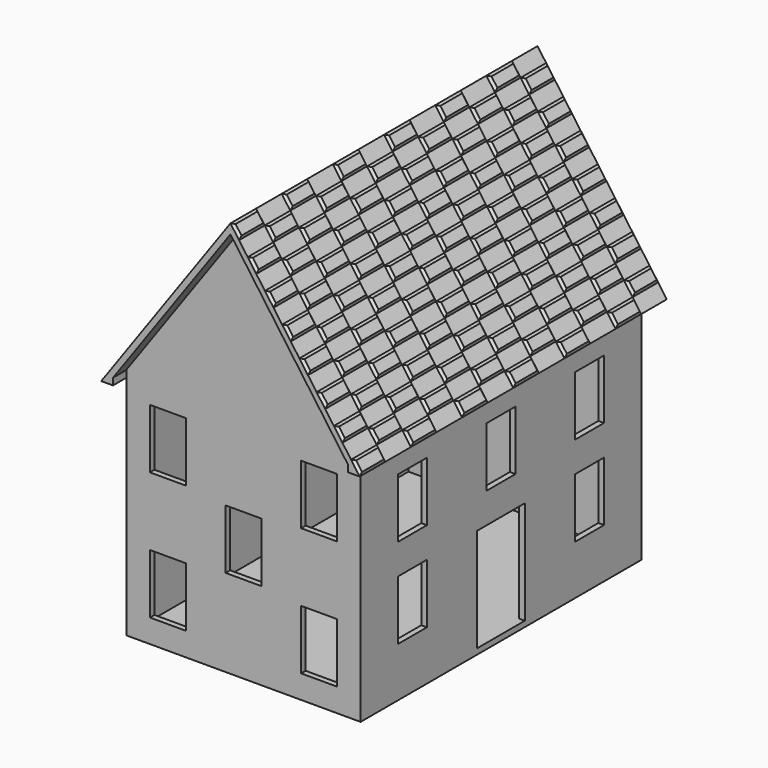
from build123d import *

# Parameters (mm, degrees)
F1_W      = 100
F1_H      = 150
F2_DEPTH  = 100
F3_T      = -2.4
F5_DEPTH  = 2.4
F7_DEPTH  = 2.4
F8_W      = 15.4
F8_H      = 25.4
F9_DEPTH  = 2.4
F10_W     = 15.4
F10_H     = 25.4
F10_W_2   = 25.4
F10_H_2   = 44.2
F11_DEPTH = 2.4
F15_DEPTH = 164
F16_W     = 13.66666672
F16_H     = 6.330327
F17_DEPTH = 1
F17_TAPER = 45
F16_W_2   = 13.6666666
F16_H_2   = 6.333333
F18_DEPTH = 1
F18_TAPER = 45


# Not quite as in the source:
# - ends of sketch curves that miss each other by under 0.0002 mm in the source are joined


with BuildPart() as f2:
    # F1 (on Top) → F2 (new body)
    with BuildSketch(Plane.XY):
        Rectangle(F1_W, F1_H)
    extrude(amount=F2_DEPTH)

    # F3
    f3_openings = [f2.faces().sort_by_distance(p)[0] for p in [
        (0, 0, 100),
    ]]
    offset(amount=F3_T, openings=f3_openings)

    # F4 (on face) → F5 (join)
    with BuildSketch(Plane.XZ.offset(75)):
        Polygon((0, 170), (-50, 100), (50, 100), align=None)
    extrude(amount=-F5_DEPTH)

    # F6 (on face) → F7 (join)
    with BuildSketch(Plane(origin=(0, 75, 0), x_dir=(-1, 0, 0), z_dir=(0, 1, 0))):
        Polygon((-50, 100), (50, 100), (0, 170), align=None)
    extrude(amount=-F7_DEPTH)

    # F8 (on face) → F9 (cut, through all)
    with BuildSketch(Plane.XZ.offset(75)):
        with Locations((-32.3, 77.3)):
            Rectangle(F8_W, F8_H)
        with Locations((32.3, 77.3)):
            Rectangle(F8_W, F8_H)
        with Locations((0, 50)):
            Rectangle(F8_W, F8_H)
        with Locations((32.3, 22.7)):
            Rectangle(F8_W, F8_H)
        with Locations((-32.3, 22.7)):
            Rectangle(F8_W, F8_H)
    extrude(amount=-F9_DEPTH, mode=Mode.SUBTRACT)

    # F10 (on face) → F11 (cut, through all)
    with BuildSketch(Plane.YZ.offset(50)):
        with Locations((-47.3, 72.3)):
            Rectangle(F10_W, F10_H)
        with Locations((47.3, 72.3)):
            Rectangle(F10_W, F10_H)
        with Locations((-47.3, 33.9)):
            Rectangle(F10_W, F10_H)
        with Locations((47.3, 33.9)):
            Rectangle(F10_W, F10_H)
        with Locations((0, 72.3)):
            Rectangle(F10_W, F10_H)
        with Locations((0, 24.5)):
            Rectangle(F10_W_2, F10_H_2)
    extrude(amount=-F11_DEPTH, mode=Mode.SUBTRACT)


with BuildPart() as f15:
    # F14 (on offset) → F15 (new body)
    with BuildSketch(Plane.XZ.offset(82)):
        Polygon((0, 174.1291161282), (-55.2176284033, 96.8244363635), (-50.2, 96.8244363635), (-50.2, 99.72), (-50, 100), (0, 170), (50, 100), (50.2, 99.72), (50.2, 96.8244363635), (55.2176284033, 96.8244363635), align=None)
    extrude(amount=-F15_DEPTH)

    # F16 (on face) → F17 (join)
    with BuildSketch(Plane(origin=(82.3583657363, 0, 58.8274040974), x_dir=(0, 1, 0), z_dir=(0.8137334712, 0, 0.5812381937))):
        Polygon((-68.3333334, 97.3693571051), (-68.3333334, 91.0400501051), (-68.3333334, 91.0390301051), (-54.66666668, 91.0390301051), (-54.66666668, 91.0400501051), (-54.66666668, 97.3693571051), align=None)
        Polygon((-68.3333334, 84.7053571051), (-68.3333334, 78.3763901051), (-68.3333334, 78.3750301051), (-54.66666668, 78.3750301051), (-54.66666668, 78.3763901051), (-54.66666668, 84.7053571051), align=None)
        Polygon((-68.3333334, 72.0413571051), (-68.3333334, 65.7127301051), (-68.3333334, 65.7110301051), (-54.66666668, 65.7110301051), (-54.66666668, 65.7127301051), (-54.66666668, 72.0413571051), align=None)
        Polygon((-68.3333334, 59.3773571051), (-68.3333334, 53.0490701051), (-68.3333334, 53.0470301051), (-54.66666668, 53.0470301051), (-54.66666668, 53.0490701051), (-54.66666668, 59.3773571051), align=None)
        with Locations((-34.16666704, 132.1961936051)):
            Rectangle(F16_W, F16_H)
        Polygon((-41.0000004, 122.6973571051), (-41.0000004, 116.3673701051), (-41.00000008, 116.3670301051), (-27.33333368, 116.3670301051), (-27.33333336, 116.3673701051), (-27.33333368, 122.6973571051), align=None)
        Polygon((-41.0000004, 110.0333571051), (-41.0000004, 103.7037101051), (-41.00000008, 103.7030301051), (-27.33333368, 103.7030301051), (-27.33333336, 103.7037101051), (-27.33333368, 110.0333571051), align=None)
        Polygon((-41.0000004, 97.3693571051), (-41.0000004, 91.0400501051), (-41.00000008, 91.0390301051), (-27.33333368, 91.0390301051), (-27.33333336, 91.0400501051), (-27.33333368, 97.3693571051), align=None)
        Polygon((-41.0000004, 84.7053571051), (-41.0000004, 78.3763901051), (-41.00000008, 78.3750301051), (-27.33333368, 78.3750301051), (-27.33333336, 78.3763901051), (-27.33333368, 84.7053571051), align=None)
        Polygon((-41.0000004, 72.0413571051), (-41.0000004, 65.7127301051), (-41.00000008, 65.7110301051), (-27.33333368, 65.7110301051), (-27.33333336, 65.7127301051), (-27.33333368, 72.0413571051), align=None)
        Polygon((-41.0000004, 59.3773571051), (-41.0000004, 53.0490701051), (-41.00000008, 53.0470301051), (-27.33333368, 53.0470301051), (-27.33333336, 53.0490701051), (-27.33333368, 59.3773571051), align=None)
        with Locations((-6.83333404, 132.1961936051)):
            Rectangle(F16_W, F16_H)
        Polygon((-13.6666674, 122.6973571051), (-13.6666674, 116.3673701051), (-13.66666676, 116.3670301051), (-6.8e-07, 116.3670301051), (-4e-08, 116.3673701051), (-6.8e-07, 122.6973571051), align=None)
        Polygon((-13.6666674, 110.0333571051), (-13.6666674, 103.7037101051), (-13.66666676, 103.7030301051), (-6.8e-07, 103.7030301051), (-4e-08, 103.7037101051), (-6.8e-07, 110.0333571051), align=None)
        Polygon((-13.6666674, 97.3693571051), (-13.6666674, 91.0400501051), (-13.66666676, 91.0390301051), (-6.8e-07, 91.0390301051), (-4e-08, 91.0400501051), (-6.8e-07, 97.3693571051), align=None)
        Polygon((-13.6666674, 84.7053571051), (-13.6666674, 78.3763901051), (-13.66666676, 78.3750301051), (-6.8e-07, 78.3750301051), (-4e-08, 78.3763901051), (-6.8e-07, 84.7053571051), align=None)
        Polygon((-13.6666674, 72.0413571051), (-13.6666674, 65.7127301051), (-13.66666676, 65.7110301051), (-6.8e-07, 65.7110301051), (-4e-08, 65.7127301051), (-6.8e-07, 72.0413571051), align=None)
        Polygon((-13.6666674, 59.3773571051), (-13.6666674, 53.0490701051), (-13.66666676, 53.0470301051), (-6.8e-07, 53.0470301051), (-4e-08, 53.0490701051), (-6.8e-07, 59.3773571051), align=None)
        with Locations((20.49999896, 132.1961936051)):
            Rectangle(F16_W, F16_H)
        Polygon((13.6666656, 122.6973571051), (13.6666656, 116.3673701051), (13.66666656, 116.3670301051), (27.33333232, 116.3670301051), (27.33333328, 116.3673701051), (27.33333232, 122.6973571051), align=None)
        Polygon((13.6666656, 110.0333571051), (13.6666656, 103.7037101051), (13.66666656, 103.7030301051), (27.33333232, 103.7030301051), (27.33333328, 103.7037101051), (27.33333232, 110.0333571051), align=None)
        Polygon((13.6666656, 97.3693571051), (13.6666656, 91.0400501051), (13.66666656, 91.0390301051), (27.33333232, 91.0390301051), (27.33333328, 91.0400501051), (27.33333232, 97.3693571051), align=None)
        Polygon((13.6666656, 84.7053571051), (13.6666656, 78.3763901051), (13.66666656, 78.3750301051), (27.33333232, 78.3750301051), (27.33333328, 78.3763901051), (27.33333232, 84.7053571051), align=None)
        Polygon((13.6666656, 72.0413571051), (13.6666656, 65.7127301051), (13.66666656, 65.7110301051), (27.33333232, 65.7110301051), (27.33333328, 65.7127301051), (27.33333232, 72.0413571051), align=None)
        Polygon((27.33333328, 53.0470301051), (27.33333328, 53.0490701051), (27.33333232, 59.3773571051), (13.6666656, 59.3773571051), (13.6666656, 53.0490701051), (13.66666656, 53.0470301051), align=None)
        with Locations((47.83333196, 132.1961936051)):
            Rectangle(F16_W, F16_H)
        Polygon((54.6666666, 116.3670301051), (54.6666666, 116.3673701051), (54.66666532, 122.6973571051), (40.9999986, 122.6973571051), (40.9999986, 116.3673701051), (40.99999988, 116.3670301051), align=None)
        Polygon((54.6666666, 103.7030301051), (54.6666666, 103.7037101051), (54.66666532, 110.0333571051), (40.9999986, 110.0333571051), (40.9999986, 103.7037101051), (40.99999988, 103.7030301051), align=None)
        Polygon((54.6666666, 91.0390301051), (54.6666666, 91.0400501051), (54.66666532, 97.3693571051), (40.9999986, 97.3693571051), (40.9999986, 91.0400501051), (40.99999988, 91.0390301051), align=None)
        Polygon((54.6666666, 78.3750301051), (54.6666666, 78.3763901051), (54.66666532, 84.7053571051), (40.9999986, 84.7053571051), (40.9999986, 78.3763901051), (40.99999988, 78.3750301051), align=None)
        Polygon((54.6666666, 65.7110301051), (54.6666666, 65.7127301051), (54.66666532, 72.0413571051), (40.9999986, 72.0413571051), (40.9999986, 65.7127301051), (40.99999988, 65.7110301051), align=None)
        Polygon((54.6666666, 53.0470301051), (54.6666666, 53.0490701051), (54.66666532, 59.3773571051), (40.9999986, 59.3773571051), (40.9999986, 53.0490701051), (40.99999988, 53.0470301051), align=None)
        with Locations((-61.50000004, 132.1961936051)):
            Rectangle(F16_W, F16_H)
        Polygon((-68.3333334, 110.0333571051), (-68.3333334, 103.7037101051), (-68.3333334, 103.7030301051), (-54.66666668, 103.7030301051), (-54.66666668, 103.7037101051), (-54.66666668, 110.0333571051), align=None)
        Polygon((-68.3333334, 122.6973571051), (-68.3333334, 116.3673701051), (-68.3333334, 116.3670301051), (-54.66666668, 116.3670301051), (-54.66666668, 116.3673701051), (-54.66666668, 122.6973571051), align=None)
        Polygon((68.3333316, 53.0470301051), (81.99999832, 53.0470301051), (81.99999832, 59.3773571051), (68.3333316, 59.3773571051), (68.3333316, 53.0490701051), align=None)
        Polygon((68.3333316, 65.7110301051), (81.99999832, 65.7110301051), (81.99999832, 72.0413571051), (68.3333316, 72.0413571051), (68.3333316, 65.7127301051), align=None)
        Polygon((81.99999832, 78.3750301051), (81.99999832, 84.7053571051), (68.3333316, 84.7053571051), (68.3333316, 78.3763901051), (68.3333332, 78.3750301051), align=None)
        Polygon((81.99999832, 91.0390301051), (81.99999832, 97.3693571051), (68.3333316, 97.3693571051), (68.3333316, 91.0400501051), (68.3333332, 91.0390301051), align=None)
        Polygon((81.99999832, 103.7030301051), (81.99999832, 110.0333571051), (68.3333316, 110.0333571051), (68.3333316, 103.7037101051), (68.3333332, 103.7030301051), align=None)
        Polygon((81.99999832, 116.3670301051), (81.99999832, 122.6973571051), (68.3333316, 122.6973571051), (68.3333316, 116.3673701051), (68.3333332, 116.3670301051), align=None)
        with Locations((75.16666496, 132.1961936051)):
            Rectangle(F16_W, F16_H)
    extrude(amount=F17_DEPTH, taper=F17_TAPER)

    # F16 (on face) → F18 (join)
    with BuildSketch(Plane(origin=(82.3583657363, 0, 58.8274040974), x_dir=(0, 1, 0), z_dir=(0.8137334712, 0, 0.5812381937))):
        with Locations((-75.1666667, 138.5280236051)):
            Rectangle(F16_W_2, F16_H_2)
        with Locations((-75.1666667, 125.8643636051)):
            Rectangle(F16_W_2, F16_H_2)
        Polygon((-68.3333334, 116.3673701051), (-82, 116.3673701051), (-82, 110.0340371051), (-68.3333334, 110.0340371051), (-68.3333334, 116.3670301051), align=None)
        Polygon((-68.3333334, 103.7037101051), (-82, 103.7037101051), (-82, 97.3703771051), (-68.3333334, 97.3703771051), (-68.3333334, 103.7030301051), align=None)
        Polygon((-68.3333334, 91.0400501051), (-82, 91.0400501051), (-82, 84.7067171051), (-68.3333334, 84.7067171051), (-68.3333334, 91.0390301051), align=None)
        Polygon((-68.3333334, 78.3763901051), (-82, 78.3763901051), (-82, 72.0430571051), (-68.3333334, 72.0430571051), (-68.3333334, 78.3750301051), align=None)
        Polygon((-68.3333334, 65.7127301051), (-82, 65.7127301051), (-82, 59.3793971051), (-68.3333334, 59.3793971051), (-68.3333334, 65.7110301051), align=None)
        Polygon((-68.3333334, 53.0490701051), (-82, 53.0490701051), (-82, 46.7157371051), (-68.3333334, 46.7157371051), (-68.3333334, 53.0470301051), align=None)
        with Locations((-47.83333338, 138.5280236051)):
            Rectangle(F16_W_2, F16_H_2)
        with Locations((-47.83333338, 125.8643636051)):
            Rectangle(F16_W_2, F16_H_2)
        with Locations((-20.50000006, 125.8643636051)):
            Rectangle(F16_W_2, F16_H_2)
        with Locations((-20.50000006, 138.5280236051)):
            Rectangle(F16_W_2, F16_H_2)
        with Locations((6.83333326, 138.5280236051)):
            Rectangle(F16_W_2, F16_H_2)
        with Locations((6.83333326, 125.8643636051)):
            Rectangle(F16_W_2, F16_H_2)
        with Locations((34.16666658, 138.5280236051)):
            Rectangle(F16_W_2, F16_H_2)
        with Locations((34.16666658, 125.8643636051)):
            Rectangle(F16_W_2, F16_H_2)
        with Locations((61.4999999, 138.5280236051)):
            Rectangle(F16_W_2, F16_H_2)
        with Locations((61.4999999, 125.8643636051)):
            Rectangle(F16_W_2, F16_H_2)
        Polygon((-54.66666668, 116.3673701051), (-54.66666668, 116.3670301051), (-54.66666668, 110.0340371051), (-41.00000008, 110.0340371051), (-41.00000008, 116.3670301051), (-41.00000008, 116.3673701051), align=None)
        Polygon((-27.33333336, 116.3673701051), (-27.33333336, 116.3670301051), (-27.33333336, 110.0340371051), (-13.66666676, 110.0340371051), (-13.66666676, 116.3670301051), (-13.66666676, 116.3673701051), align=None)
        Polygon((-4e-08, 116.3673701051), (-4e-08, 116.3670301051), (-4e-08, 110.0340371051), (13.66666656, 110.0340371051), (13.66666656, 116.3670301051), (13.66666656, 116.3673701051), align=None)
        Polygon((27.33333328, 116.3673701051), (27.33333328, 116.3670301051), (27.33333328, 110.0340371051), (40.99999988, 110.0340371051), (40.99999988, 116.3670301051), (40.99999988, 116.3673701051), align=None)
        Polygon((68.3333332, 116.3670301051), (68.3333332, 116.3673701051), (54.6666666, 116.3673701051), (54.6666666, 116.3670301051), (54.6666666, 110.0340371051), (68.3333332, 110.0340371051), align=None)
        Polygon((68.3333332, 103.7030301051), (68.3333332, 103.7037101051), (54.6666666, 103.7037101051), (54.6666666, 103.7030301051), (54.6666666, 97.3703771051), (68.3333332, 97.3703771051), align=None)
        Polygon((27.33333328, 103.7037101051), (27.33333328, 103.7030301051), (27.33333328, 97.3703771051), (40.99999988, 97.3703771051), (40.99999988, 103.7030301051), (40.99999988, 103.7037101051), align=None)
        Polygon((-4e-08, 103.7037101051), (-4e-08, 103.7030301051), (-4e-08, 97.3703771051), (13.66666656, 97.3703771051), (13.66666656, 103.7030301051), (13.66666656, 103.7037101051), align=None)
        Polygon((-27.33333336, 103.7037101051), (-27.33333336, 103.7030301051), (-27.33333336, 97.3703771051), (-13.66666676, 97.3703771051), (-13.66666676, 103.7030301051), (-13.66666676, 103.7037101051), align=None)
        Polygon((-54.66666668, 103.7037101051), (-54.66666668, 103.7030301051), (-54.66666668, 97.3703771051), (-41.00000008, 97.3703771051), (-41.00000008, 103.7030301051), (-41.00000008, 103.7037101051), align=None)
        Polygon((-54.66666668, 91.0400501051), (-54.66666668, 91.0390301051), (-54.66666668, 84.7067171051), (-41.00000008, 84.7067171051), (-41.00000008, 91.0390301051), (-41.00000008, 91.0400501051), align=None)
        Polygon((-27.33333336, 91.0400501051), (-27.33333336, 91.0390301051), (-27.33333336, 84.7067171051), (-13.66666676, 84.7067171051), (-13.66666676, 91.0390301051), (-13.66666676, 91.0400501051), align=None)
        Polygon((-4e-08, 91.0400501051), (-4e-08, 91.0390301051), (-4e-08, 84.7067171051), (13.66666656, 84.7067171051), (13.66666656, 91.0390301051), (13.66666656, 91.0400501051), align=None)
        Polygon((27.33333328, 91.0400501051), (27.33333328, 91.0390301051), (27.33333328, 84.7067171051), (40.99999988, 84.7067171051), (40.99999988, 91.0390301051), (40.99999988, 91.0400501051), align=None)
        Polygon((68.3333332, 91.0390301051), (68.3333332, 91.0400501051), (54.6666666, 91.0400501051), (54.6666666, 91.0390301051), (54.6666666, 84.7067171051), (68.3333332, 84.7067171051), align=None)
        Polygon((-54.66666668, 78.3763901051), (-54.66666668, 78.3750301051), (-54.66666668, 72.0430571051), (-41.00000008, 72.0430571051), (-41.00000008, 78.3750301051), (-41.00000008, 78.3763901051), align=None)
        Polygon((-27.33333336, 78.3763901051), (-27.33333336, 78.3750301051), (-27.33333336, 72.0430571051), (-13.66666676, 72.0430571051), (-13.66666676, 78.3750301051), (-13.66666676, 78.3763901051), align=None)
        Polygon((-4e-08, 78.3763901051), (-4e-08, 78.3750301051), (-4e-08, 72.0430571051), (13.66666656, 72.0430571051), (13.66666656, 78.3750301051), (13.66666656, 78.3763901051), align=None)
        Polygon((27.33333328, 78.3763901051), (27.33333328, 78.3750301051), (27.33333328, 72.0430571051), (40.99999988, 72.0430571051), (40.99999988, 78.3750301051), (40.99999988, 78.3763901051), align=None)
        Polygon((68.3333332, 78.3750301051), (68.3333332, 78.3763901051), (54.6666666, 78.3763901051), (54.6666666, 78.3750301051), (54.6666666, 72.0430571051), (68.3333332, 72.0430571051), align=None)
        Polygon((-54.66666668, 65.7127301051), (-54.66666668, 65.7110301051), (-54.66666668, 59.3793971051), (-41.00000008, 59.3793971051), (-41.00000008, 65.7110301051), (-41.00000008, 65.7127301051), align=None)
        Polygon((-27.33333336, 65.7127301051), (-27.33333336, 65.7110301051), (-27.33333336, 59.3793971051), (-13.66666676, 59.3793971051), (-13.66666676, 65.7110301051), (-13.66666676, 65.7127301051), align=None)
        Polygon((-4e-08, 65.7127301051), (-4e-08, 65.7110301051), (-4e-08, 59.3793971051), (13.66666656, 59.3793971051), (13.66666656, 65.7110301051), (13.66666656, 65.7127301051), align=None)
        Polygon((40.99999988, 59.3793971051), (40.99999988, 65.7110301051), (40.99999988, 65.7127301051), (27.33333328, 65.7127301051), (27.33333328, 65.7110301051), (27.33333328, 59.3793971051), align=None)
        Polygon((68.3333332, 59.3793971051), (68.3333332, 65.7110301051), (68.3333332, 65.7127301051), (54.6666666, 65.7127301051), (54.6666666, 65.7110301051), (54.6666666, 59.3793971051), align=None)
        Polygon((68.3333332, 46.7157371051), (68.3333332, 53.0470301051), (68.3333332, 53.0490701051), (54.6666666, 53.0490701051), (54.6666666, 53.0470301051), (54.6666666, 46.7157371051), align=None)
        Polygon((40.99999988, 46.7157371051), (40.99999988, 53.0470301051), (40.99999988, 53.0490701051), (27.33333328, 53.0490701051), (27.33333328, 53.0470301051), (27.33333328, 46.7157371051), align=None)
        Polygon((-4e-08, 53.0490701051), (-4e-08, 53.0470301051), (-4e-08, 46.7157371051), (13.66666656, 46.7157371051), (13.66666656, 53.0470301051), (13.66666656, 53.0490701051), align=None)
        Polygon((-27.33333336, 53.0490701051), (-27.33333336, 53.0470301051), (-27.33333336, 46.7157371051), (-13.66666676, 46.7157371051), (-13.66666676, 53.0470301051), (-13.66666676, 53.0490701051), align=None)
        Polygon((-54.66666668, 53.0490701051), (-54.66666668, 53.0470301051), (-54.66666668, 46.7157371051), (-41.00000008, 46.7157371051), (-41.00000008, 53.0470301051), (-41.00000008, 53.0490701051), align=None)
    extrude(amount=F18_DEPTH, taper=F18_TAPER)


solid = Compound([f2.part, f15.part])
